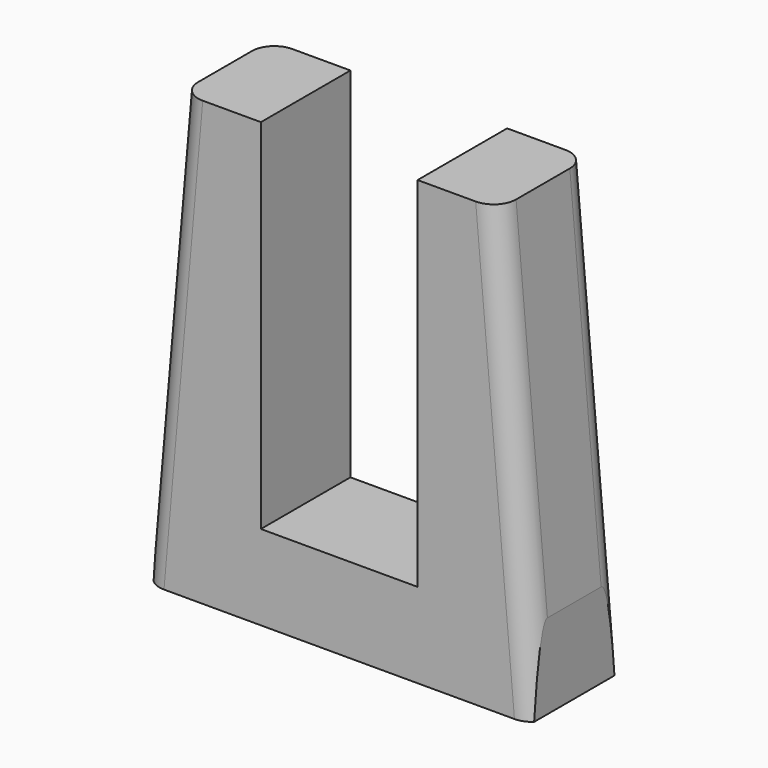
from build123d import *

# Parameters (mm, degrees)
F1_DEPTH    = 2.5
F2_T1_DEPTH = 15.5305666052
F2_T3_DEPTH = 15.5305666052


# Not quite as in the source:
# - a fillet or chamfer that OpenCascade refuses, or shapes differently, is made with other operations: its cross-section is extruded or revolved along the edge and cut away or added


with BuildPart() as f1:
    # F0 (on Front) → F1 (new body)
    with BuildSketch(Plane.XZ):
        Polygon((0, -1.894692351), (0, 0), (-1.75, 0), (-4.25, 0), (-4.25, -1.894692351), align=None)
        Polygon((1.75, 0), (0, 0), (0, -1.894692351), (4.25, -1.894692351), (4.25, 0), align=None)
        Polygon((-4.25, 0), (-1.75, 0), (-1.75, 8), (-3.55, 8), align=None)
        Polygon((1.75, 8), (1.75, 0), (4.25, 0), (3.55, 8), align=None)
    extrude(amount=F1_DEPTH)

    # F2: fillet of radius 0.5 on 4 edges, made by hand

    # F2_s2 → F2_t1 (cut)
    with BuildSketch(Plane(origin=(0.5770852674, 0, -6.5952601994), x_dir=(0, 1, 0), z_dir=(-0.0871669503, 0, 0.9961937175))):
        with BuildLine():
            ThreePointArc((-2, -4.2338232994), (-2.3535533906, -4.08737669), (-2.5, -3.7338232994))
            Line((-2.5, -3.7338232994), (-2.5, -4.2338232994))
            Line((-2.5, -4.2338232994), (-2, -4.2338232994))
        make_face()
        with BuildLine():
            ThreePointArc((-0.5, -4.2338232994), (-0.1464466094, -4.08737669), (0, -3.7338232994))
            Line((0, -3.7338232994), (0, -4.2338232994))
            Line((0, -4.2338232994), (-0.5, -4.2338232994))
        make_face()
    extrude(amount=F2_T1_DEPTH, mode=Mode.SUBTRACT)

    # F2_s4 → F2_t3 (cut)
    with BuildSketch(Plane(origin=(0.7766668597, 0, 8.8761926818), x_dir=(0, 1, 0), z_dir=(-0.0871669503, 0, -0.9961937175))):
        with BuildLine():
            ThreePointArc((-2, -4.2338232994), (-2.3535533906, -4.08737669), (-2.5, -3.7338232994))
            Line((-2.5, -3.7338232994), (-2.5, -4.2338232994))
            Line((-2.5, -4.2338232994), (-2, -4.2338232994))
        make_face()
        with BuildLine():
            ThreePointArc((-0.5, -4.2338232994), (-0.1464466094, -4.08737669), (0, -3.7338232994))
            Line((0, -3.7338232994), (0, -4.2338232994))
            Line((0, -4.2338232994), (-0.5, -4.2338232994))
        make_face()
    extrude(amount=F2_T3_DEPTH, mode=Mode.SUBTRACT)


solid = f1.part
